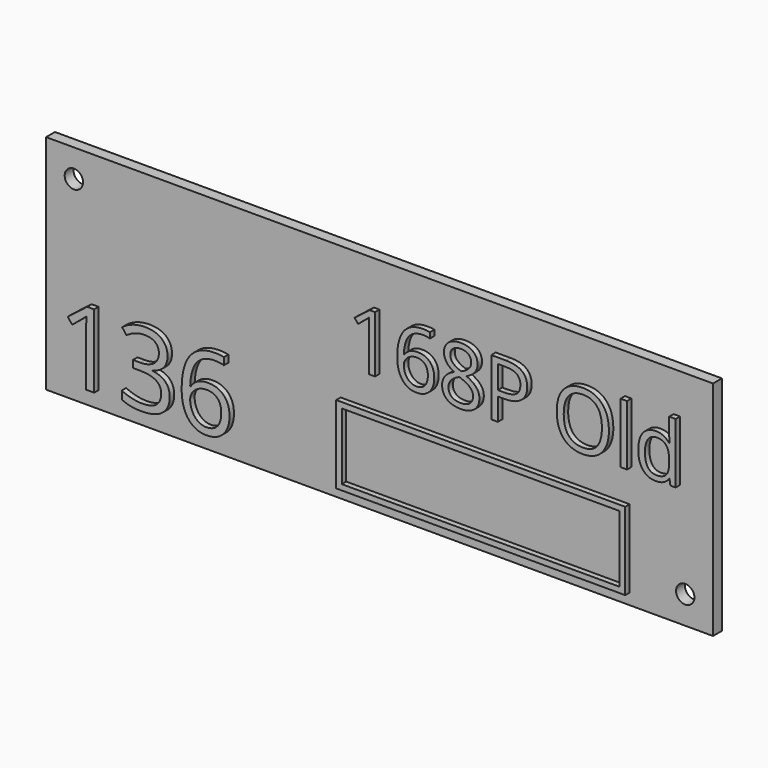
from build123d import *

# Parameters (mm, degrees)
F0_W         = 120
F0_H         = 40
F1_DEPTH     = 2
F3_D         = 3.3
F4_TEXT_SIZE = 14.2841200759
F5_DEPTH     = 1
F6_TEXT_SIZE = 18.4837545126
F7_DEPTH     = 1
F8_W         = 52
F8_H         = 14
F8_W_2       = 49.99999962
F8_H_2       = 11.99999962
F9_DEPTH     = 1


# Not quite as in the source:
# - Text() gives the source's letters only with a copy of the font that has no kerning and outlines rounded to 1/6400 em; it was checked with that copy


with BuildPart() as f1:
    # F0 (on Front) → F1 (new body)
    with BuildSketch(Plane.XZ):
        Rectangle(F0_W, F0_H)
    extrude(amount=F1_DEPTH)

    # F3 (through all)
    with Locations(Plane.XZ.offset(2)):
        with Locations((-55, 15), (55, -15)):
            Hole(F3_D / 2)

    # F4 (on face) → F5 (join)
    with BuildSketch(Plane.XZ.offset(2)):
        with Locations((-5, 2)):
            Text('168P Old', F4_TEXT_SIZE, font='Open Sans', text_align=(TextAlign.LEFT, TextAlign.BOTTOM))
    extrude(amount=F5_DEPTH)

    # F6 (on face) → F7 (join)
    with BuildSketch(Plane.XZ.offset(2)):
        with Locations((-57, -17)):
            Text('136', F6_TEXT_SIZE, font='Open Sans', text_align=(TextAlign.LEFT, TextAlign.BOTTOM))
    extrude(amount=F7_DEPTH)

    # F8 (on face) → F9 (join)
    with BuildSketch(Plane.XZ.offset(2)):
        with Locations((19, -11)):
            Rectangle(F8_W, F8_H)
        with Locations((19, -11)):
            Rectangle(F8_W_2, F8_H_2, mode=Mode.SUBTRACT)
    extrude(amount=F9_DEPTH)


solid = f1.part
